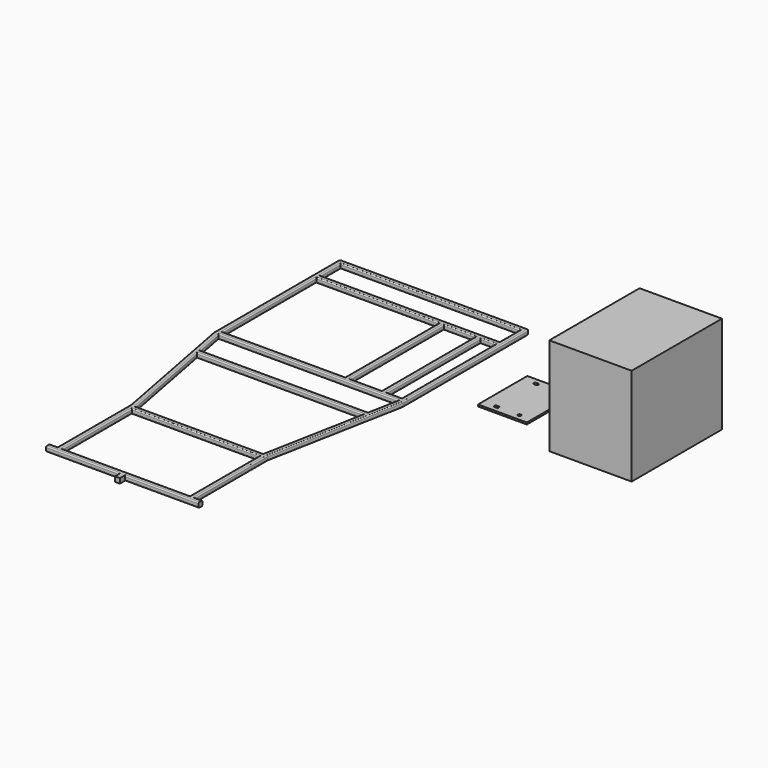
from build123d import *

# Parameters (mm, degrees)
F0_W     = 25
F0_H     = 16
F0_W_2   = 16
F0_H_2   = 20
F0_H_3   = 384
F0_W_3   = 418
F1_DEPTH = 16
F2_R     = 3.5
F3_W     = 270
F3_H     = 370
F4_DEPTH = 320
F5_W     = 160
F5_H     = 202
F5_R     = 5
F6_DEPTH = 6


# Not quite as in the source:
# - a feature names something its author has since deleted; it is built from what else it names


with BuildPart() as f1:
    # F0 (on Top) → F1 (new body)
    with BuildSketch(Plane.XY):
        Polygon((209, -589.2307258319), (225, -589.2307258319), (225, -573.2307258319), (225, -273.2307258319), (310, 173.2307258319), (310, 589.2307258319), (294, 589.2307258319), (-294, 589.2307258319), (-310, 589.2307258319), (-310, 173.2307258319), (-225, -273.2307258319), (-225, -573.2307258319), (-225, -589.2307258319), (-209, -589.2307258319), (-8, -589.2307258319), (8, -589.2307258319), align=None)
        Polygon((244, 573.2307258319), (294, 573.2307258319), (294, 189.2307258319), (294, 173.2307258319), (274.9614022256, 73.2307258319), (271.9152265817, 57.2307258319), (209, -273.2307258319), (209, -289.2307258319), (209, -573.2307258319), (-209, -573.2307258319), (-209, -289.2307258319), (-209, -273.2307258319), (-271.9152265817, 57.2307258319), (-274.9614022256, 73.2307258319), (-294, 173.2307258319), (-294, 189.2307258319), (-294, 573.2307258319), (108, 573.2307258319), (124, 573.2307258319), (228, 573.2307258319), align=None, mode=Mode.SUBTRACT)
        with Locations((237.5, -581.2307258319)):
            Rectangle(F0_W, F0_H)
        with Locations((0, -599.2307258319)):
            Rectangle(F0_W_2, F0_H_2)
        with BuildLine():
            Line((294, 589.2307258319), (310, 589.2307258319))
            Line((310, 589.2307258319), (310, 684.2307258319))
            ThreePointArc((310, 684.2307258319), (308.5355339059, 687.7662597378), (305, 689.2307258319))
            Line((305, 689.2307258319), (-305, 689.2307258319))
            ThreePointArc((-305, 689.2307258319), (-308.5355339059, 687.7662597378), (-310, 684.2307258319))
            Line((-310, 684.2307258319), (-310, 589.2307258319))
            Line((-310, 589.2307258319), (-294, 589.2307258319))
            Line((-294, 589.2307258319), (-294, 673.2307258319))
            Line((-294, 673.2307258319), (294, 673.2307258319))
            Line((294, 673.2307258319), (294, 589.2307258319))
        make_face()
        with Locations((-237.5, -581.2307258319)):
            Rectangle(F0_W, F0_H)
        with Locations((236, 381.2307258319)):
            Rectangle(F0_W_2, F0_H_3)
        Polygon((294, 173.2307258319), (294, 189.2307258319), (244, 189.2307258319), (228, 189.2307258319), (124, 189.2307258319), (108, 189.2307258319), (-294, 189.2307258319), (-294, 173.2307258319), align=None)
        with Locations((116, 381.2307258319)):
            Rectangle(F0_W_2, F0_H_3)
        Polygon((271.9152265817, 57.2307258319), (274.9614022256, 73.2307258319), (-274.9614022256, 73.2307258319), (-271.9152265817, 57.2307258319), align=None)
        with Locations((0, -281.2307258319)):
            Rectangle(F0_W_3, F0_H)
    extrude(amount=F1_DEPTH)

    # F2
    f2_edges = [f1.edges().sort_by_distance(p)[0] for p in [
        (0, -573.230726, 16),
        (-93, 573.230726, 16),
        (0, 589.230726, 16),
        (0, 673.230726, 16),
        (0, 689.230726, 16),
        (310, 428.730726, 16),
        (294, 631.230726, 16),
        (-294, 631.230726, 16),
        (-310, 428.730726, 16),
        (0, 689.230726, 0),
        (0, -573.230726, 0),
        (0, 673.230726, 0),
        (-294, 381.230726, 16),
        (294, 381.230726, 16),
        (-240.457613, -108, 16),
        (240.457613, -108, 16),
        (0, -273.230726, 16),
        (0, -289.230726, 16),
        (-267.5, -50, 16),
        (-209, -431.230726, 16),
        (209, -431.230726, 16),
        (267.5, -50, 16),
        (0, -289.230726, 0),
        (0, -273.230726, 0),
        (240.457613, -108, 0),
        (267.5, -50, 0),
        (-240.457613, -108, 0),
        (-225, -423.230726, 0),
        (-267.5, -50, 0),
        (294, 381.230726, 0),
        (-294, 381.230726, 0),
        (-93, 573.230726, 0),
        (0, 589.230726, 0),
        (294, 631.230726, 0),
        (310, 428.730726, 0),
        (-294, 631.230726, 0),
        (209, -431.230726, 0),
        (0, 173.230726, 16),
        (-93, 189.230726, 16),
        (108, 381.230726, 16),
        (124, 381.230726, 16),
        (228, 381.230726, 16),
        (244, 381.230726, 16),
        (108, 381.230726, 0),
        (228, 381.230726, 0),
        (244, 381.230726, 0),
        (124, 381.230726, 0),
        (0, 73.230726, 16),
        (0, 57.230726, 16),
        (0, 73.230726, 0),
        (0, 57.230726, 0),
        (0, 173.230726, 0),
        (-93, 189.230726, 0),
        (-237.5, -573.230726, 16),
        (-129, -589.230726, 0),
        (-237.5, -573.230726, 0),
        (-129, -589.230726, 16),
        (237.5, -573.230726, 16),
        (129, -589.230726, 16),
        (129, -589.230726, 0),
        (237.5, -573.230726, 0),
        (225, -423.230726, 0),
        (225, -423.230726, 16),
        (-225, -423.230726, 16),
        (-209, -431.230726, 0),
        (308.535534, 687.76626, 0),
        (308.535534, 687.76626, 16),
        (-308.535534, 687.76626, 0),
        (-308.535534, 687.76626, 16),
        (-310, 428.730726, 0),
        (-284.480701, 123.230726, 0),
        (-284.480701, 123.230726, 16),
        (284.480701, 123.230726, 0),
        (284.480701, 123.230726, 16),
        (176, 573.230726, 0),
        (176, 573.230726, 16),
        (176, 189.230726, 16),
        (269, 573.230726, 0),
        (269, 573.230726, 16),
        (269, 189.230726, 16),
    ]]
    fillet(f2_edges, radius=F2_R)


with BuildPart() as f4:
    # F3 (on Top) → F4 (new body)
    with BuildSketch(Plane.XY):
        with Locations((888.8288272917, 403.0536437035)):
            Rectangle(F3_W, F3_H)
    extrude(amount=F4_DEPTH)


with BuildPart() as f6:
    # F5 (on Top) → F6 (new body)
    with BuildSketch(Plane.XY):
        with Locations((536.598880291, 398.6082916385)):
            Rectangle(F5_W, F5_H)
        with BuildLine():
            ThreePointArc((494.098880291, 317.6082916385), (495.5633463851, 321.1438255445), (499.098880291, 322.6082916385))
            Line((499.098880291, 322.6082916385), (504.098880291, 322.6082916385))
            ThreePointArc((504.098880291, 322.6082916385), (507.6344141969, 321.1438255445), (509.098880291, 317.6082916385))
            ThreePointArc((509.098880291, 317.6082916385), (507.6344141969, 314.0727577326), (504.098880291, 312.6082916385))
            Line((504.098880291, 312.6082916385), (499.098880291, 312.6082916385))
            ThreePointArc((499.098880291, 312.6082916385), (495.5633463851, 314.0727577326), (494.098880291, 317.6082916385))
        make_face(mode=Mode.SUBTRACT)
        with Locations((576.598880291, 317.6082916385)):
            Circle(F5_R, mode=Mode.SUBTRACT)
        with BuildLine():
            ThreePointArc((494.098880291, 479.6082916385), (495.5633463851, 483.1438255445), (499.098880291, 484.6082916385))
            Line((499.098880291, 484.6082916385), (504.098880291, 484.6082916385))
            ThreePointArc((504.098880291, 484.6082916385), (507.6344141969, 483.1438255445), (509.098880291, 479.6082916385))
            ThreePointArc((509.098880291, 479.6082916385), (507.6344141969, 476.0727577326), (504.098880291, 474.6082916385))
            Line((504.098880291, 474.6082916385), (499.098880291, 474.6082916385))
            ThreePointArc((499.098880291, 474.6082916385), (495.5633463851, 476.0727577326), (494.098880291, 479.6082916385))
        make_face(mode=Mode.SUBTRACT)
        with Locations((576.598880291, 479.6082916385)):
            Circle(F5_R, mode=Mode.SUBTRACT)
    extrude(amount=F6_DEPTH)


solid = Compound([f1.part, f4.part, f6.part])
